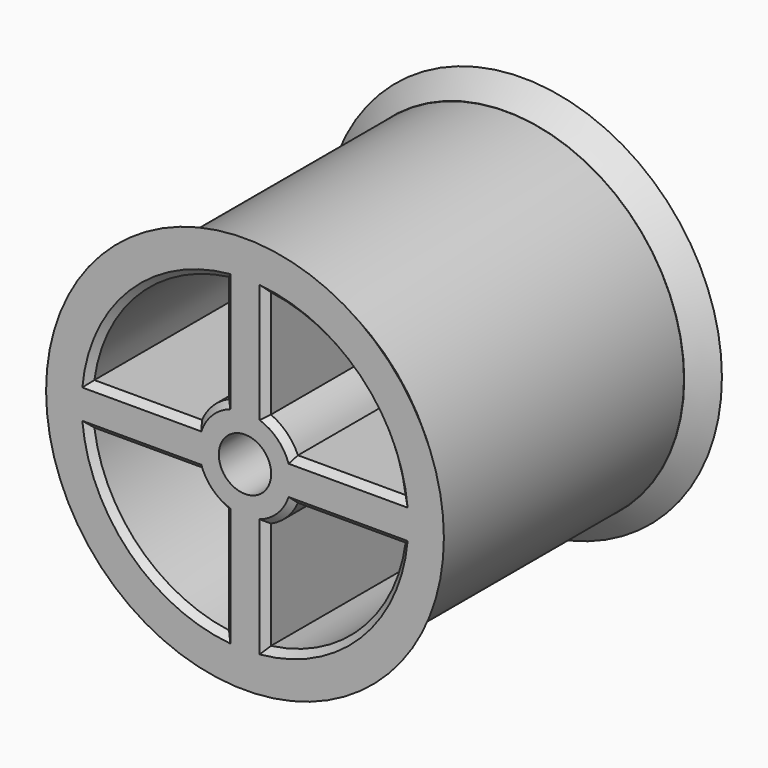
from build123d import *

# Parameters (mm, degrees)
F0_R     = 84.89324665
F1_DEPTH = 166
F2_R     = 95
F2_R_2   = 84.89324665
F3_DEPTH = 10
F4_R     = 95
F4_R_2   = 84.89324665
F5_DEPTH = 10
F6_SIZE  = 9.99999
F7_R     = 12.5
F8_DEPTH = 166.001
F9_SIZE  = 3


# Not quite as in the source:
# - a fillet or chamfer is up to 0.001 mm smaller than in the source, because OpenCascade refuses the exact size


with BuildPart() as f1:
    # F0 (on Front) → F1 (new body)
    with BuildSketch(Plane.XZ):
        Circle(F0_R)
    extrude(amount=F1_DEPTH)

    # F2 (on face) → F3 (join)
    with BuildSketch(Plane(origin=(0, 0, 0), x_dir=(-1, 0, 0), z_dir=(0, 1, 0))):
        Circle(F2_R)
        Circle(F2_R_2, mode=Mode.SUBTRACT)
    extrude(amount=-F3_DEPTH)

    # F4 (on face) → F5 (join)
    with BuildSketch(Plane.XZ.offset(166)):
        Circle(F4_R)
        Circle(F4_R_2, mode=Mode.SUBTRACT)
    extrude(amount=-F5_DEPTH)

    # F6 (size 10 in the source; OpenCascade refuses exactly that, so slightly less here)
    f6_edges = [f1.edges().sort_by_distance(p)[0] for p in [
        (95, -10, 0),
        (-95, -156, 0),
    ]]
    chamfer(f6_edges, length=F6_SIZE)

    # F7 (on face) → F8 (cut, through all)
    with BuildSketch(Plane(origin=(0, 0, 0), x_dir=(-1, 0, 0), z_dir=(0, 1, 0))):
        with BuildLine():
            Line((-10, 22.9128784748), (-10, 74.3303437366))
            ThreePointArc((-10, 74.3303437366), (-53.033008589, 53.033008589), (-74.3303437366, 10))
            Line((-74.3303437366, 10), (-22.9128784748, 10))
            ThreePointArc((-22.9128784748, 10), (-17.6776695297, 17.6776695297), (-10, 22.9128784748))
        make_face()
        with BuildLine():
            Line((22.9128784748, 10), (74.3303437366, 10))
            ThreePointArc((74.3303437366, 10), (53.033008589, 53.033008589), (10, 74.3303437366))
            Line((10, 74.3303437366), (10, 22.9128784748))
            ThreePointArc((10, 22.9128784748), (17.6776695297, 17.6776695297), (22.9128784748, 10))
        make_face()
        with BuildLine():
            ThreePointArc((-74.3303437366, -10), (-53.033008589, -53.033008589), (-10, -74.3303437366))
            Line((-10, -74.3303437366), (-10, -22.9128784748))
            ThreePointArc((-10, -22.9128784748), (-17.6776695297, -17.6776695297), (-22.9128784748, -10))
            Line((-22.9128784748, -10), (-74.3303437366, -10))
        make_face()
        with BuildLine():
            ThreePointArc((10, -74.3303437366), (53.033008589, -53.033008589), (74.3303437366, -10))
            Line((74.3303437366, -10), (22.9128784748, -10))
            ThreePointArc((22.9128784748, -10), (17.6776695297, -17.6776695297), (10, -22.9128784748))
            Line((10, -22.9128784748), (10, -74.3303437366))
        make_face()
        Circle(F7_R)
    extrude(amount=-F8_DEPTH, mode=Mode.SUBTRACT)

    # F9
    f9_edges = [f1.edges().sort_by_distance(p)[0] for p in [
        (-53.033009, -166, 53.033009),
        (-10, -166, 48.621611),
        (-48.621611, -166, 10),
        (-17.67767, -166, 17.67767),
        (53.033009, -166, 53.033009),
        (48.621611, -166, 10),
        (17.67767, -166, 17.67767),
        (10, -166, 48.621611),
        (48.621611, -166, -10),
        (53.033009, -166, -53.033009),
        (17.67767, -166, -17.67767),
        (10, -166, -48.621611),
        (-10, -166, -48.621611),
        (-17.67767, -166, -17.67767),
        (-48.621611, -166, -10),
        (-53.033009, -166, -53.033009),
        (-53.033009, 0, 53.033009),
        (-10, 0, 48.621611),
        (-17.67767, 0, 17.67767),
        (-48.621611, 0, 10),
        (-53.033009, 0, -53.033009),
        (-48.621611, 0, -10),
        (-17.67767, 0, -17.67767),
        (-10, 0, -48.621611),
        (10, 0, 48.621611),
        (53.033009, 0, 53.033009),
        (17.67767, 0, 17.67767),
        (48.621611, 0, 10),
        (17.67767, 0, -17.67767),
        (10, 0, -48.621611),
        (48.621611, 0, -10),
        (53.033009, 0, -53.033009),
    ]]
    chamfer(f9_edges, length=F9_SIZE)


solid = f1.part
